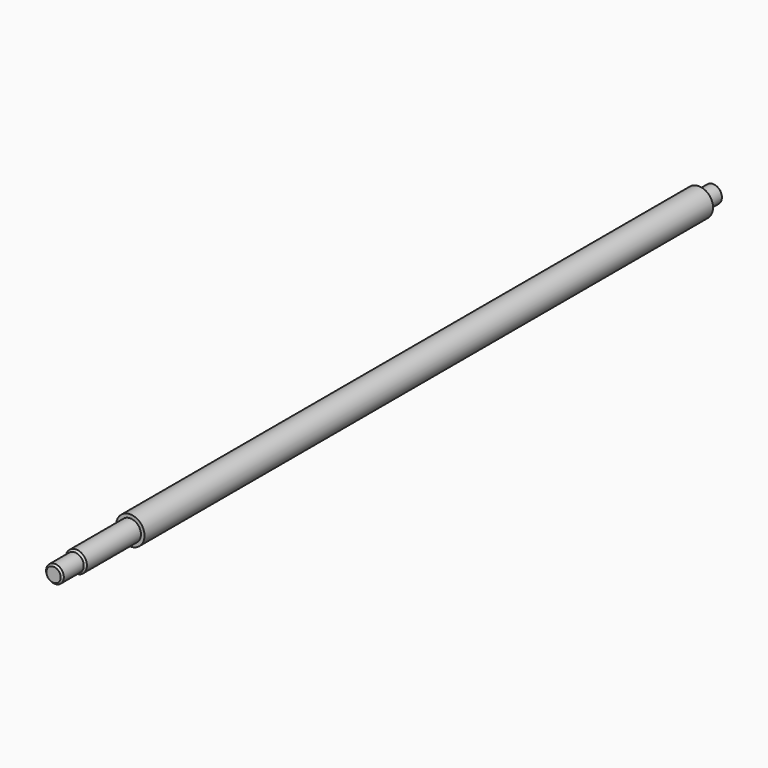
from build123d import *

# Parameters (mm, degrees)
F2_SIZE = 0.99999


# Not quite as in the source:
# - a fillet or chamfer is up to 0.001 mm smaller than in the source, because OpenCascade refuses the exact size


with BuildPart() as f1:
    # F0 (on Right) → F1 (revolve)
    with BuildSketch(Plane.YZ):
        Polygon((0, 5), (0, 0), (465, 0), (465, 5), (454, 5), (454, 8), (54, 8), (54, 6), (15, 6), (15, 5), align=None)
    revolve(axis=Axis((0, 344.1624132916, 0), (0, 1, 0)))

    # F2 (size 1 in the source; OpenCascade refuses exactly that, so slightly less here)
    f2_edges = [f1.edges().sort_by_distance(p)[0] for p in [
        (0, 0, -5),
        (0, 15, -6),
        (0, 465, -5),
    ]]
    chamfer(f2_edges, length=F2_SIZE)


solid = f1.part
